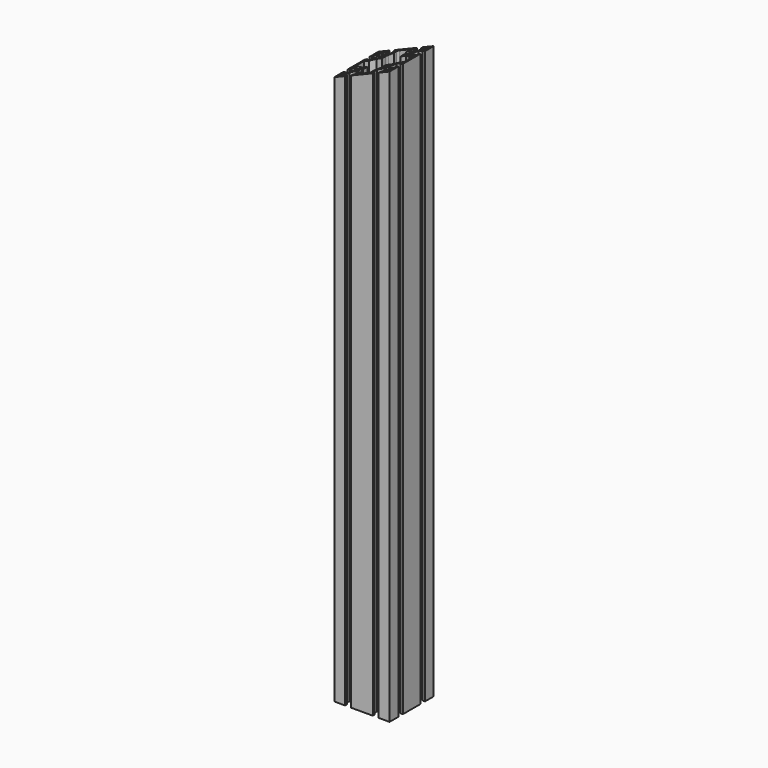
from build123d import *

# Parameters (mm, degrees)
F0_R          = 3
F0_R_2        = 2.5
F1_DEPTH      = 621.5
F2_R          = 2
F3_R          = 7
F6_DEPTH      = 30
F6_DEPTH_BACK = 30


# Not quite as in the source:
# - a feature names something its author has since deleted; it is built from what else it names


with BuildPart() as f1:
    # F0 (on Top) → F1 (new body)
    with BuildSketch(Plane.XY):
        with BuildLine():
            Line((18.15, -30), (30, -30))
            Line((30, -30), (30, -18.15))
            Line((30, -18.15), (27.5, -18.15))
            Line((27.5, -18.15), (27.5, -20.15))
            Line((27.5, -20.15), (21.5477069044, -20.15))
            ThreePointArc((21.5477069044, -20.15), (19.5, -15), (21.5477069044, -9.85))
            Line((21.5477069044, -9.85), (27.5, -9.85))
            Line((27.5, -9.85), (27.5, -11.85))
            Line((27.5, -11.85), (30, -11.85))
            Line((30, -11.85), (30, 11.85))
            Line((30, 11.85), (27.5, 11.85))
            Line((27.5, 11.85), (27.5, 9.85))
            Line((27.5, 9.85), (21.5477069044, 9.85))
            ThreePointArc((21.5477069044, 9.85), (19.5, 15), (21.5477069044, 20.15))
            Line((21.5477069044, 20.15), (27.5, 20.15))
            Line((27.5, 20.15), (27.5, 18.15))
            Line((27.5, 18.15), (30, 18.15))
            Line((30, 18.15), (30, 30))
            Line((30, 30), (18.15, 30))
            Line((18.15, 30), (18.15, 27.5))
            Line((18.15, 27.5), (20.15, 27.5))
            Line((20.15, 27.5), (20.15, 21.5477069044))
            ThreePointArc((20.15, 21.5477069044), (15, 19.5), (9.85, 21.5477069044))
            Line((9.85, 21.5477069044), (9.85, 27.5))
            Line((9.85, 27.5), (11.85, 27.5))
            Line((11.85, 27.5), (11.85, 30))
            Line((11.85, 30), (-11.85, 30))
            Line((-11.85, 30), (-11.85, 27.5))
            Line((-11.85, 27.5), (-9.85, 27.5))
            Line((-9.85, 27.5), (-9.85, 21.5477069044))
            ThreePointArc((-9.85, 21.5477069044), (-15, 19.5), (-20.15, 21.5477069044))
            Line((-20.15, 21.5477069044), (-20.15, 27.5))
            Line((-20.15, 27.5), (-18.15, 27.5))
            Line((-18.15, 27.5), (-18.15, 30))
            Line((-18.15, 30), (-30, 30))
            Line((-30, 30), (-30, 18.15))
            Line((-30, 18.15), (-27.5, 18.15))
            Line((-27.5, 18.15), (-27.5, 20.15))
            Line((-27.5, 20.15), (-21.5477069044, 20.15))
            ThreePointArc((-21.5477069044, 20.15), (-19.5, 15), (-21.5477069044, 9.85))
            Line((-21.5477069044, 9.85), (-27.5, 9.85))
            Line((-27.5, 9.85), (-27.5, 11.85))
            Line((-27.5, 11.85), (-30, 11.85))
            Line((-30, 11.85), (-30, -11.85))
            Line((-30, -11.85), (-27.5, -11.85))
            Line((-27.5, -11.85), (-27.5, -9.85))
            Line((-27.5, -9.85), (-21.5477069044, -9.85))
            ThreePointArc((-21.5477069044, -9.85), (-19.5, -15), (-21.5477069044, -20.15))
            Line((-21.5477069044, -20.15), (-27.5, -20.15))
            Line((-27.5, -20.15), (-27.5, -18.15))
            Line((-27.5, -18.15), (-30, -18.15))
            Line((-30, -18.15), (-30, -30))
            Line((-30, -30), (-18.15, -30))
            Line((-18.15, -30), (-18.15, -27.5))
            Line((-18.15, -27.5), (-20.15, -27.5))
            Line((-20.15, -27.5), (-20.15, -21.5477069044))
            ThreePointArc((-20.15, -21.5477069044), (-15, -19.5), (-9.85, -21.5477069044))
            Line((-9.85, -21.5477069044), (-9.85, -27.5))
            Line((-9.85, -27.5), (-11.85, -27.5))
            Line((-11.85, -27.5), (-11.85, -30))
            Line((-11.85, -30), (11.85, -30))
            Line((11.85, -30), (11.85, -27.5))
            Line((11.85, -27.5), (9.85, -27.5))
            Line((9.85, -27.5), (9.85, -21.5477069044))
            ThreePointArc((9.85, -21.5477069044), (15, -19.5), (20.15, -21.5477069044))
            Line((20.15, -21.5477069044), (20.15, -27.5))
            Line((20.15, -27.5), (18.15, -27.5))
            Line((18.15, -27.5), (18.15, -30))
        make_face()
        with Locations((-25, -25)):
            Circle(F0_R, mode=Mode.SUBTRACT)
        with Locations((-15, -15)):
            Circle(F0_R_2, mode=Mode.SUBTRACT)
        with Locations((25, -25)):
            Circle(F0_R, mode=Mode.SUBTRACT)
        with Locations((15, -15)):
            Circle(F0_R_2, mode=Mode.SUBTRACT)
        with Locations((-25, 25)):
            Circle(F0_R, mode=Mode.SUBTRACT)
        with Locations((-15, 15)):
            Circle(F0_R_2, mode=Mode.SUBTRACT)
        Polygon((-7, 22), (-7, 27.5), (0, 27.5), (7, 27.5), (7, 22), (10, 16), (10, 10), (16, 10), (22, 7), (27.5, 7), (27.5, 0), (27.5, -7), (22, -7), (16, -10), (10, -10), (10, -16), (7, -22), (7, -27.5), (0, -27.5), (-7, -27.5), (-7, -22), (-10, -16), (-10, -10), (-16, -10), (-22, -7), (-27.5, -7), (-27.5, 0), (-27.5, 7), (-22, 7), (-16, 10), (-10, 10), (-10, 16), align=None, mode=Mode.SUBTRACT)
        with Locations((15, 15)):
            Circle(F0_R_2, mode=Mode.SUBTRACT)
        with Locations((25, 25)):
            Circle(F0_R, mode=Mode.SUBTRACT)
    extrude(amount=F1_DEPTH)

    # F2
    f2_edges = [f1.edges().sort_by_distance(p)[0] for p in [
        (-7, 27.5, 310.75),
        (7, 27.5, 310.75),
    ]]
    fillet(f2_edges, radius=F2_R)

    # F3
    f3_edges = [f1.edges().sort_by_distance(p)[0] for p in [
        (-10, 16, 310.75),
        (10, 16, 310.75),
    ]]
    fillet(f3_edges, radius=F3_R)

    # F5 (on Front) → F6 (cut, two sides)
    with BuildSketch(Plane.XZ) as f6_sk:
        Polygon((30, 621.5), (-11.184961555, 720.929292752), (-183.3312368923, 649.6239707953), (-142.1462753372, 550.1946780433), align=None)
    extrude(amount=F6_DEPTH, mode=Mode.SUBTRACT)
    extrude(f6_sk.sketch, amount=-F6_DEPTH_BACK, mode=Mode.SUBTRACT)


solid = f1.part
